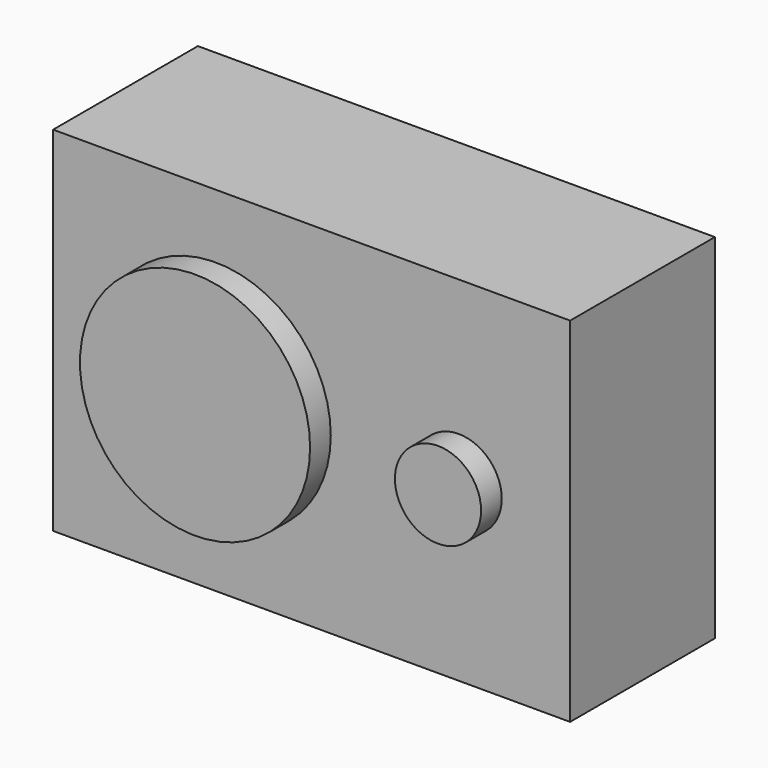
from build123d import *

# Parameters (mm, degrees)
F0_W     = 60
F0_H     = 41
F1_DEPTH = 21
F2_R     = 13.3531025353
F2_R_2   = 5
F3_DEPTH = 3


# Not quite as in the source:
# - a feature names something its author has since deleted; it is built from what else it names


with BuildPart() as f1:
    # F0 (on Front) → F1 (new body)
    with BuildSketch(Plane.XZ):
        Rectangle(F0_W, F0_H)
    extrude(amount=F1_DEPTH)

    # F2 (on face) → F3 (join)
    with BuildSketch(Plane.XZ.offset(21)):
        with Locations((-11.1307431944, -0.2782683878)):
            Circle(F2_R)
        with Locations((17.0671385713, -0.2782683878)):
            Circle(F2_R_2)
    extrude(amount=F3_DEPTH)


solid = f1.part
